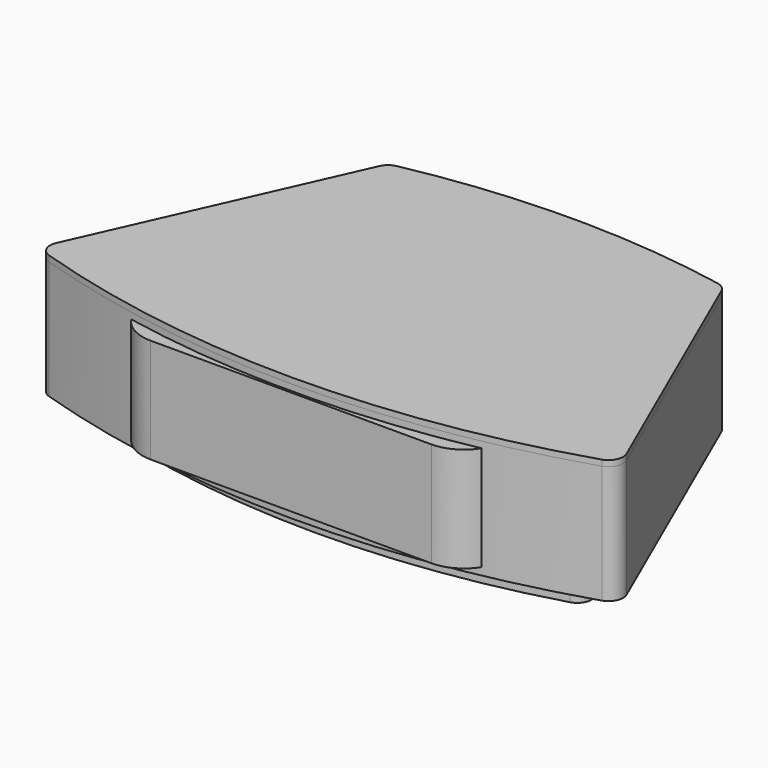
from build123d import *

# Parameters (mm, degrees)
F1_DEPTH    = 51.435
F3_DEPTH    = 10.16
F5_DEPTH    = 2.54
F6_R        = 6.35
F6_2_R      = 6.35
F6_3_R      = 6.35
F7_W        = 151.9614458084
F7_H        = 45.4733071383
F8_DEPTH    = 71.374
F9_T1_DEPTH = 120.0136733796
F9_T3_DEPTH = 120.9407803299


# Not quite as in the source:
# - a fillet or chamfer that OpenCascade refuses, or shapes differently, is made with other operations: its cross-section is extruded or revolved along the edge and cut away or added


with BuildPart() as f1:
    # F0 (on Top) → F1 (new body)
    with BuildSketch(Plane.XY):
        with BuildLine():
            ThreePointArc((73.2254907489, 73.2552930713), (0.5247097559, 80.2488736751), (-72.0931589603, 72.4412575364))
            Line((-72.0931589603, 72.4412575364), (-126.6336739063, -49.6643856168))
            ThreePointArc((-126.6336739063, -49.6643856168), (0.1613423228, -70.4870011046), (126.956358552, -49.6643856168))
            Line((126.956358552, -49.6643856168), (73.2254907489, 73.2552930713))
        make_face()
    extrude(amount=-F1_DEPTH)

    # F6
    f6_edges = [f1.edges().sort_by_distance(p)[0] for p in [
        (-126.633674, -49.664386, -25.7175),
        (126.956359, -49.664386, -25.7175),
        (73.225491, 73.255293, -25.7175),
        (-72.093159, 72.441258, -25.7175),
    ]]
    fillet(f6_edges, radius=F6_R)

    # F7 (on Front) → F8 (join)
    with BuildSketch(Plane.XZ):
        with Locations((0.9076371789, -25.4708082648)):
            Rectangle(F7_W, F7_H)
    extrude(amount=F8_DEPTH)

    # F9: fillet of radius 17.78 on 2 edges, made by hand

    # F9_s2 → F9_t1 (cut)
    with BuildSketch(Plane.XY.offset(-85.4776449546)):
        with BuildLine():
            ThreePointArc((-75.0730857253, -63.2830532058), (-68.6460806292, -69.2208961409), (-60.1650124771, -71.374))
            Line((-60.1650124771, -71.374), (-75.0730857253, -71.374))
            Line((-75.0730857253, -71.374), (-75.0730857253, -63.2830532058))
        make_face()
    extrude(amount=F9_T1_DEPTH, mode=Mode.SUBTRACT)

    # F9_s4 → F9_t3 (cut)
    with BuildSketch(Plane.XY.offset(-85.9411984297)):
        with BuildLine():
            ThreePointArc((76.8883600831, -62.9915964801), (70.427337124, -69.1377715085), (61.7948654448, -71.374))
            Line((61.7948654448, -71.374), (76.8883600831, -71.374))
            Line((76.8883600831, -71.374), (76.8883600831, -62.9915964801))
        make_face()
    extrude(amount=F9_T3_DEPTH, mode=Mode.SUBTRACT)


with BuildPart() as f3:
    # F2 (on face) → F3 (new body)
    with BuildSketch(Plane(origin=(0, 0, -51.435), x_dir=(1, 0, 0), z_dir=(0, 0, -1))):
        with BuildLine():
            ThreePointArc((107.4105203152, 42.1924516559), (0.6039142609, 58.4204568292), (-106.2026917934, 42.1924516559))
            Line((-106.2026917934, 42.1924516559), (-60.175538063, -60.7785619795))
            ThreePointArc((-60.175538063, -60.7785619795), (0.751433894, -65.3222976326), (61.6784058511, -60.7785619795))
            Line((61.6784058511, -60.7785619795), (107.4105203152, 42.1924516559))
        make_face()
    extrude(amount=F3_DEPTH)

    # F6#2
    f6_2_edges = [f3.edges().sort_by_distance(p)[0] for p in [
        (-106.202692, -42.192452, -56.515),
        (107.41052, -42.192452, -56.515),
        (61.678406, 60.778562, -56.515),
        (-60.175538, 60.778562, -56.515),
    ]]
    fillet(f6_2_edges, radius=F6_2_R)


with BuildPart() as f5:
    # F4 (on face) → F5 (new body)
    with BuildSketch(Plane.XY):
        with BuildLine():
            ThreePointArc((-126.6336739063, -49.6643856168), (0.1613423228, -70.4870011046), (126.956358552, -49.6643856168))
            Line((126.956358552, -49.6643856168), (73.2254907489, 73.2552930713))
            ThreePointArc((73.2254907489, 73.2552930713), (0.5247097559, 80.2488736751), (-72.0931589603, 72.4412575364))
            Line((-72.0931589603, 72.4412575364), (-126.6336739063, -49.6643856168))
        make_face()
    extrude(amount=F5_DEPTH)

    # F6#3
    f6_3_edges = [f5.edges().sort_by_distance(p)[0] for p in [
        (-126.633674, -49.664386, 1.27),
        (126.956359, -49.664386, 1.27),
        (73.225491, 73.255293, 1.27),
        (-72.093159, 72.441258, 1.27),
    ]]
    fillet(f6_3_edges, radius=F6_3_R)


solid = Compound([f1.part, f3.part, f5.part])
